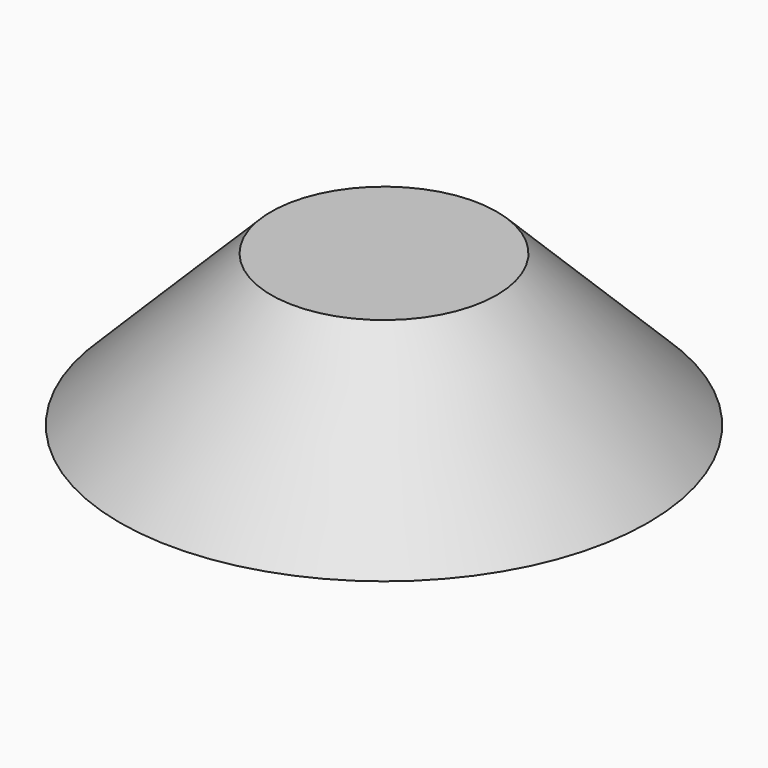
from build123d import *

# Parameters (mm, degrees)
F0_R     = 26.6102890419
F1_DEPTH = 15.24
F2_SIZE  = 15.23999


# Not quite as in the source:
# - a fillet or chamfer is up to 0.001 mm smaller than in the source, because OpenCascade refuses the exact size


with BuildPart() as f1:
    # F0 (on Top) → F1 (new body)
    with BuildSketch(Plane.XY):
        with Locations((-21.2452597916, 18.9964585006)):
            Circle(F0_R)
    extrude(amount=F1_DEPTH)

    # F2 (size 15.24 in the source; OpenCascade refuses exactly that, so slightly less here)
    f2_edges = [f1.edges().sort_by_distance(p)[0] for p in [
        (-47.855549, 18.996459, 15.24),
    ]]
    chamfer(f2_edges, length=F2_SIZE)


solid = f1.part
